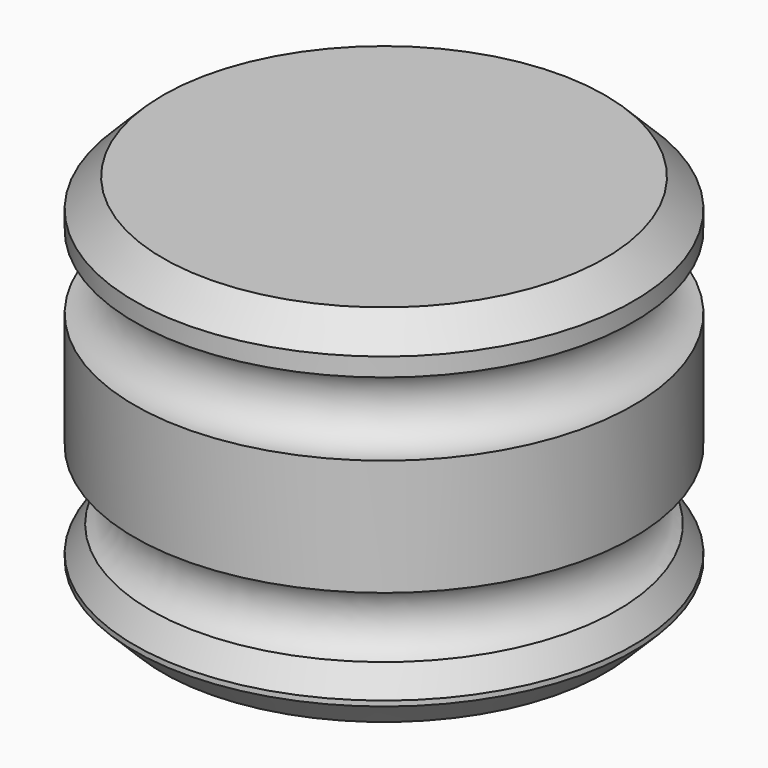
from build123d import *


# Not quite as in the source:
# - a fillet or chamfer that OpenCascade refuses, or shapes differently, is made with other operations: its cross-section is extruded or revolved along the edge and cut away or added


with BuildPart() as f1:
    # F0 (on Front) → F1 (revolve)
    with BuildSketch(Plane.XZ):
        with BuildLine():
            Line((-44.4924347103, 0), (0, 0))
            Line((0, 0), (0, 65.1155337691))
            Line((0, 65.1155337691), (-44.4924347103, 65.1155337691))
            Line((-44.4924347103, 65.1155337691), (-44.4924347103, 56.7583087614))
            ThreePointArc((-44.4924347103, 56.7583087614), (-37.9552003214, 50.2210743725), (-44.4924347103, 43.6838399837))
            Line((-44.4924347103, 43.6838399837), (-44.4924347103, 22.9257815758))
            ThreePointArc((-44.4924347103, 22.9257815758), (-37.9887534996, 16.4221003652), (-44.4924347103, 9.9184191545))
            Line((-44.4924347103, 9.9184191545), (-44.4924347103, 0))
        make_face()
    revolve(axis=Axis((0, 0, 32.5577668846), (0, 0, 1)))

    # F2: chamfer of 5.08 on 4 edges, made by hand

    # F2_s1 → F2_t2 (revolve, cut)
    with BuildSketch(Plane.XZ):
        Polygon((-39.4124347103, 65.1155337691), (-44.4924347103, 60.0355337691), (-44.4924347103, 65.1155337691), align=None)
    revolve(axis=Axis((0, 0, 65.1155337691), (0, 0, 1)), mode=Mode.SUBTRACT)

    # F2_s3 → F2_t4 (revolve, cut)
    with BuildSketch(Plane.XZ):
        with BuildLine():
            Line((-44.4924347103, 6.0117559717), (-41.6402584505, 10.5771914803))
            ThreePointArc((-41.6402584505, 10.5771914803), (-42.9562364784, 10.1024513019), (-44.4924347103, 9.9184191545))
            Line((-44.4924347103, 9.9184191545), (-44.4924347103, 6.0117559717))
        make_face()
    revolve(axis=Axis((0, 0, 9.9184191545), (0, 0, 1)), mode=Mode.SUBTRACT)

    # F2_s5 → F2_t6 (revolve, cut)
    with BuildSketch(Plane.XZ):
        Polygon((-44.4924347103, 5.08), (-39.4124347103, 0), (-44.4924347103, 0), align=None)
    revolve(axis=Axis((0, 0, 0), (0, 0, 1)), mode=Mode.SUBTRACT)


solid = f1.part
